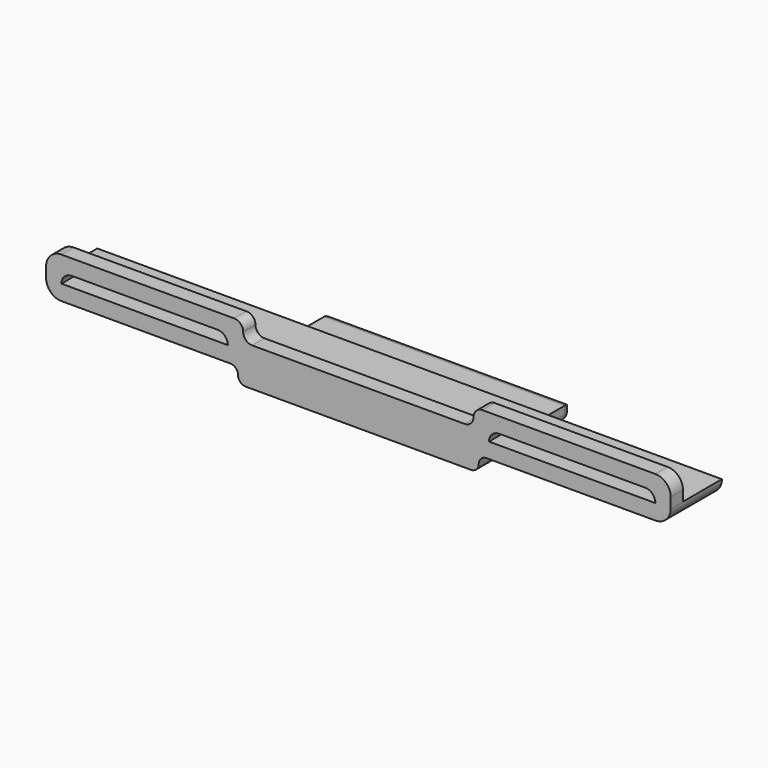
from build123d import *

# Parameters (mm, degrees)
F1_DEPTH = 6
F2_DEPTH = 25
F0_W     = 94
F0_H     = 6
F3_DEPTH = 45
F4_W     = 65
F4_H     = 4
F5_DEPTH = 25
F6_R     = 3.99999
F7_R     = 3.49999
F8_R     = 5.99999
F9_R     = 2.99999


# Not quite as in the source:
# - two fillets or chamfers of one size are made in one step
# - a fillet or chamfer is up to 0.001 mm smaller than in the source, because OpenCascade refuses the exact size


with BuildPart() as f1:
    # F0 (on Front) → F1 (new body)
    with BuildSketch(Plane.XZ):
        Polygon((-122, 22), (-122, 12), (122, 12), (122, 22), (45, 22), (45, 15), (-45, 15), (-45, 22), align=None)
    extrude(amount=-F1_DEPTH)

    # F0 (on Front) → F2 (join)
    with BuildSketch(Plane.XZ):
        Polygon((-122, 12), (-122, 6), (-47, 6), (47, 6), (122, 6), (122, 12), align=None)
    extrude(amount=-F2_DEPTH)

    # F0 (on Front) → F3 (join, through all)
    with BuildSketch(Plane.XZ):
        with Locations((0, 3)):
            Rectangle(F0_W, F0_H)
    extrude(amount=-F3_DEPTH)

    # F4 (on face) → F5 (cut)
    with BuildSketch(Plane(origin=(0, 6, 0), x_dir=(-1, 0, 0), z_dir=(0, 1, 0))):
        with Locations((83.5, 14)):
            Rectangle(F4_W, F4_H)
        with Locations((-83.5, 14)):
            Rectangle(F4_W, F4_H)
    extrude(amount=-F5_DEPTH, mode=Mode.SUBTRACT)

    # F6 (radius 4 in the source; OpenCascade refuses exactly that, so slightly less here)
    f6_edges = [f1.edges().sort_by_distance(p)[0] for p in [
        (-51, 3, 16),
        (-116, 3, 16),
        (51, 3, 16),
        (116, 3, 16),
    ]]
    fillet(f6_edges, radius=F6_R)

    # F7 (radius 3.5 in the source; OpenCascade refuses exactly that, so slightly less here)
    f7_edges = [f1.edges().sort_by_distance(p)[0] for p in [
        (-45, 3, 15),
        (-45, 3, 22),
        (45, 3, 15),
        (45, 3, 22),
    ]]
    fillet(f7_edges, radius=F7_R)

    # F8 (radius 6 in the source; OpenCascade refuses exactly that, so slightly less here)
    f8_edges = [f1.edges().sort_by_distance(p)[0] for p in [
        (-122, 3, 22),
        (122, 3, 22),
        (-122, 12.5, 6),
        (122, 12.5, 6),
    ]]
    fillet(f8_edges, radius=F8_R)

    # F9 (radius 3 in the source; OpenCascade refuses exactly that, so slightly less here)
    f9_edges = [f1.edges().sort_by_distance(p)[0] for p in [
        (47, 12.5, 6),
        (47, 22.5, 0),
        (-47, 22.5, 0),
        (-47, 12.5, 6),
        (-47, 45, 3),
        (0, 45, 0),
        (47, 45, 3),
        (0, 45, 6),
    ]]
    fillet(f9_edges, radius=F9_R)


solid = f1.part
